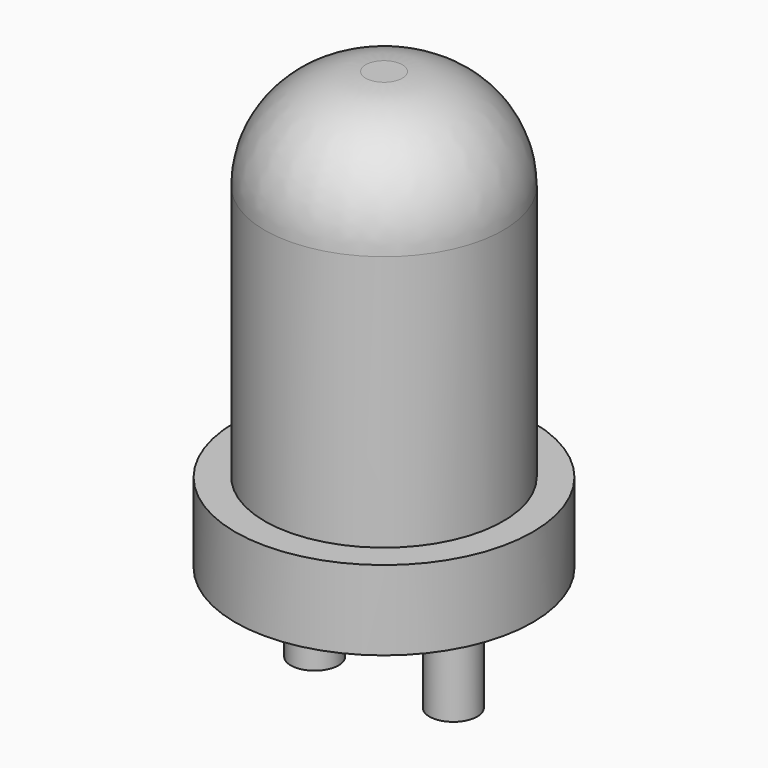
from build123d import *

# Parameters (mm, degrees)
F2_R     = 0.3
F3_DEPTH = 1.27


# Not quite as in the source:
# - a feature names something its author has since deleted; it is built from what else it names


with BuildPart() as f1:
    # F0 (on Front) → F1 (revolve)
    with BuildSketch(Plane.XZ):
        with BuildLine():
            Line((-1.87, 0), (0, 0))
            Line((0, 0), (0, 5.49))
            Line((0, 5.49), (-0.23, 5.49))
            ThreePointArc((-0.23, 5.49), (-1.1280256121, 5.1180256121), (-1.5, 4.22))
            Line((-1.5, 4.22), (-1.5, 1))
            Line((-1.5, 1), (-1.87, 1))
            Line((-1.87, 1), (-1.87, 0))
        make_face()
    revolve(axis=Axis((0, 0, 2.745), (0, 0, -1)))

    # F2 (on face) → F3 (join)
    with BuildSketch(Plane(origin=(0, 0, 0), x_dir=(1, 0, 0), z_dir=(0, 0, -1))):
        with Locations((-0.8715403965, 0)):
            Circle(F2_R)
        with Locations((0.8715403965, 0)):
            Circle(F2_R)
    extrude(amount=F3_DEPTH)


solid = f1.part
